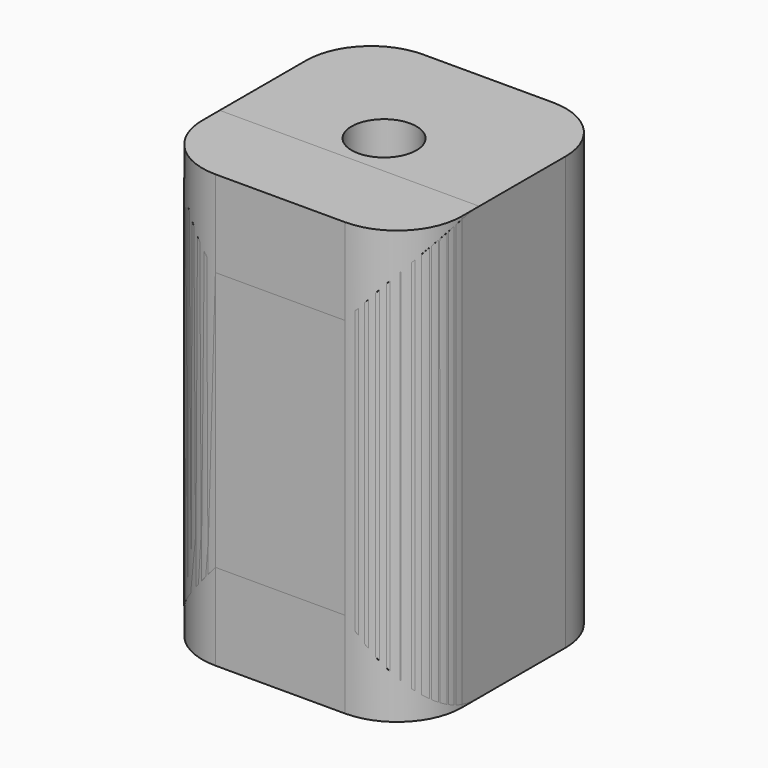
from build123d import *

# Parameters (mm, degrees)
F1_DEPTH    = 20
F2_DEPTH    = 20
F3_T1_DEPTH = 26
F4_D        = 3
F4_2_D      = 3


# Not quite as in the source:
# - a fillet or chamfer that OpenCascade refuses, or shapes differently, is made with other operations: its cross-section is extruded or revolved along the edge and cut away or added


with BuildPart() as f1:
    # F0 (on Top) → F1 (new body)
    with BuildSketch(Plane.XY):
        with BuildLine():
            ThreePointArc((6, 3), (5.1213203436, 5.1213203436), (3, 6))
            Line((3, 6), (-3, 6))
            ThreePointArc((-3, 6), (-5.1213203436, 5.1213203436), (-6, 3))
            Line((-6, 3), (-6, -3))
            ThreePointArc((-6, -3), (-5.1213203436, -5.1213203436), (-3, -6))
            Line((-3, -6), (3, -6))
            ThreePointArc((3, -6), (5.1213203436, -5.1213203436), (6, -3))
            Line((6, -3), (6, 3))
        make_face()
    extrude(amount=F1_DEPTH)

    # F4 (through all)
    with Locations(Plane(origin=(0, 0, 0), x_dir=(1, 0, 0), z_dir=(0, 0, -1))):
        with Locations((0, 0)):
            Hole(F4_D / 2)


with BuildPart() as f2:
    # F0 (on Top) → F2 (new body)
    with BuildSketch(Plane.XY):
        with BuildLine():
            ThreePointArc((6, 3), (5.1213203436, 5.1213203436), (3, 6))
            Line((3, 6), (-3, 6))
            ThreePointArc((-3, 6), (-5.1213203436, 5.1213203436), (-6, 3))
            Line((-6, 3), (-6, -3))
            ThreePointArc((-6, -3), (-5.1213203436, -5.1213203436), (-3, -6))
            Line((-3, -6), (3, -6))
            ThreePointArc((3, -6), (5.1213203436, -5.1213203436), (6, -3))
            Line((6, -3), (6, 3))
        make_face()
    extrude(amount=F2_DEPTH)

    # F3: fillet of radius 4 on 2 edges, made by hand

    # F3_s2 → F3_t1 (cut)
    with BuildSketch(Plane.YZ.offset(-13)):
        with BuildLine():
            ThreePointArc((-6, 16), (-4.8284271247, 18.8284271247), (-2, 20))
            Line((-2, 20), (-6, 20))
            Line((-6, 20), (-6, 16))
        make_face()
        with BuildLine():
            ThreePointArc((-6, 4), (-4.8284271247, 1.1715728753), (-2, 0))
            Line((-2, 0), (-6, 0))
            Line((-6, 0), (-6, 4))
        make_face()
    extrude(amount=F3_T1_DEPTH, mode=Mode.SUBTRACT)

    # F4#2 (through all)
    with Locations(Plane(origin=(0, 0, 0), x_dir=(1, 0, 0), z_dir=(0, 0, -1))):
        with Locations((0, 0)):
            Hole(F4_2_D / 2)


solid = Compound([f1.part, f2.part])
